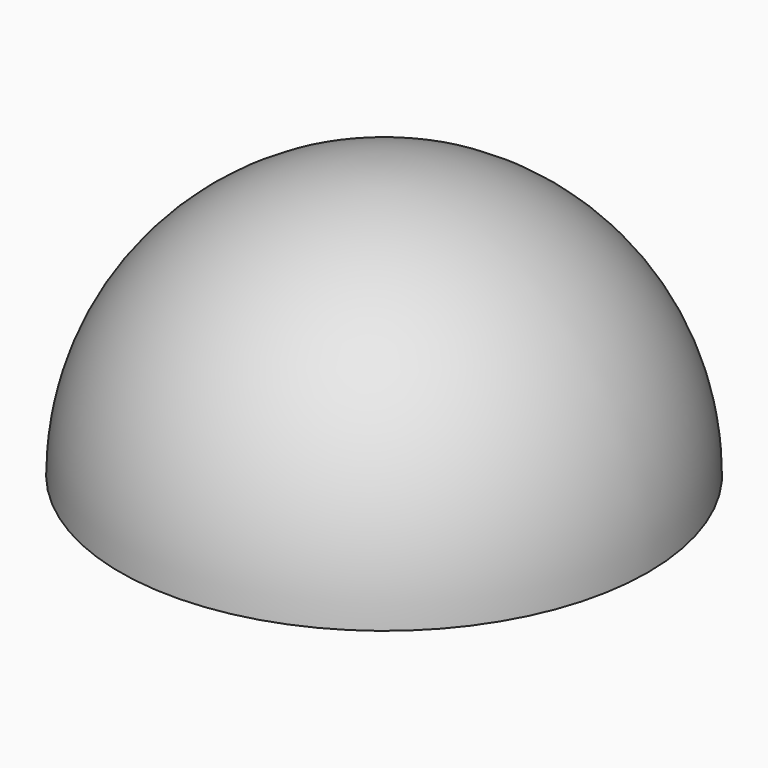
from build123d import *


# Not quite as in the source:
# - the program builds the solid bodies; features that only make, move or delete a surface that nothing else refers to are left out


with BuildPart() as f1:
    # F0 (on Front) → F1 (revolve)
    with BuildSketch(Plane.XZ):
        with BuildLine():
            Line((32, 0), (35, 0))
            ThreePointArc((35, 0), (24.7487373415, 24.7487373415), (0, 35))
            Line((0, 35), (0, 32))
            ThreePointArc((0, 32), (22.627416998, 22.627416998), (32, 0))
        make_face()
    revolve(axis=Axis((0, 0, 33.5), (0, 0, -1)))


solid = f1.part
